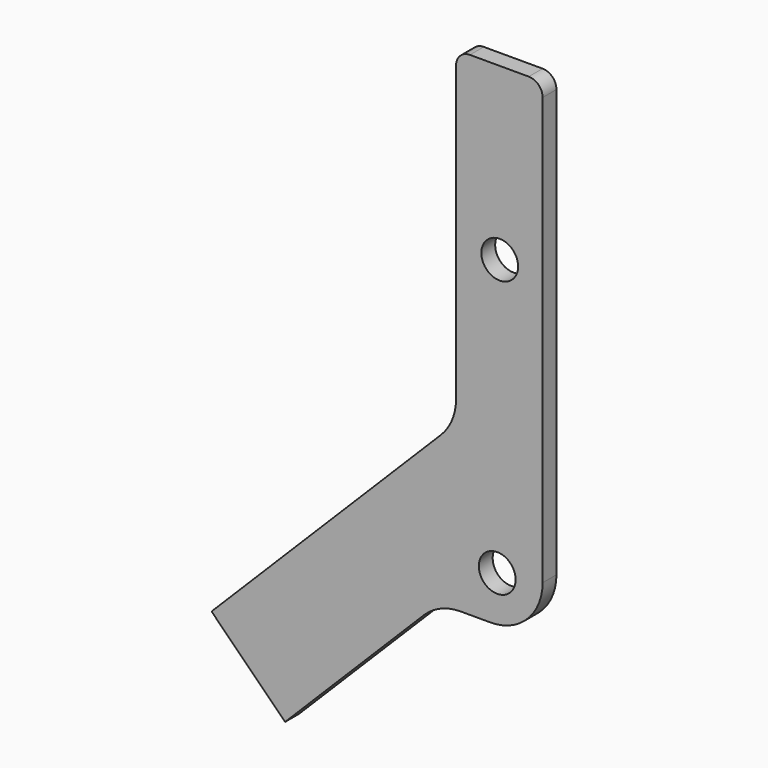
from build123d import *

# Parameters (mm, degrees)
F1_DEPTH = 6.35
F3_D     = 13.49248
F4_R     = 19.05
F5_R     = 5.08


# Not quite as in the source:
# - a feature names something its author has since deleted; it is built from what else it names


with BuildPart() as f1:
    # F0 (on Front) → F1 (new body)
    with BuildSketch(Plane.XZ):
        Polygon((37.9981123171, 180.8299914), (6.2481123171, 180.8299914), (6.2481123171, 60.2186896705), (-47.5612342455, 6.2650593709), (-83.434131954, -29.7040274954), (-56.4573168042, -56.6087007767), (-20.5844190958, -20.6396139104), (0, 0), (6.2481123171, 0), (37.9981123171, 0), (37.9981123171, 33.02), align=None)
    extrude(amount=F1_DEPTH)

    # F3 (through all)
    with Locations(Plane.XZ.offset(6.35)):
        with Locations((22.2628123171, 118.2443914), (21.3484123171, 16.8009124652)):
            Hole(F3_D / 2)

    # F4
    f4_edges = [f1.edges().sort_by_distance(p)[0] for p in [
        (6.248112, -3.175, 60.21869),
        (37.998112, -3.175, 0),
        (0, -3.175, 0),
    ]]
    fillet(f4_edges, radius=F4_R)

    # F5
    f5_edges = [f1.edges().sort_by_distance(p)[0] for p in [
        (6.248112, -3.175, 180.829991),
        (37.998112, -3.175, 180.829991),
    ]]
    fillet(f5_edges, radius=F5_R)


solid = f1.part
